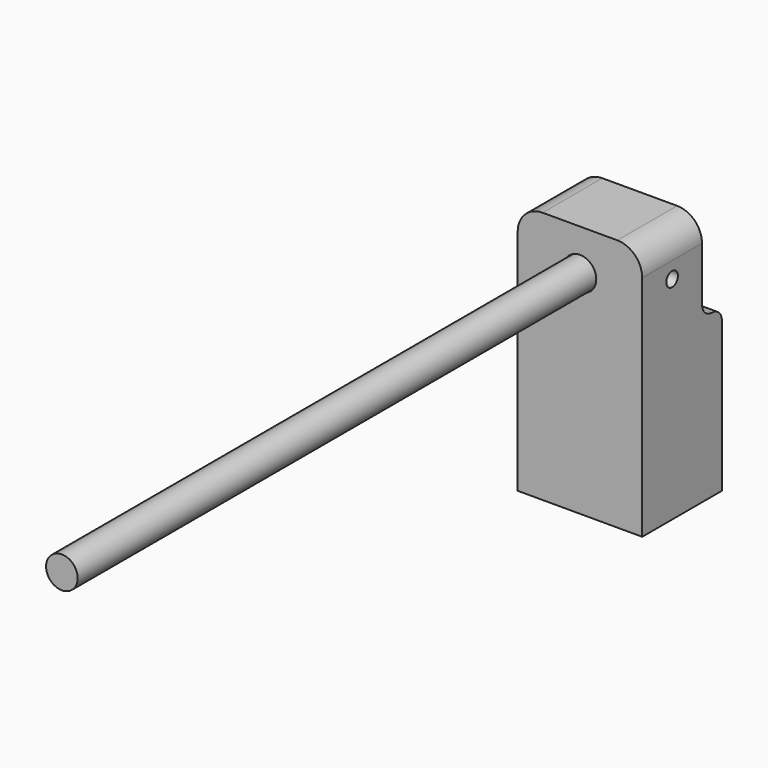
from build123d import *

# Parameters (mm, degrees)
F0_W      = 50
F0_H      = 101.55
F0_R      = 6.55
F1_DEPTH  = 40
F3_R      = 2.9
F4_DEPTH  = 50.001
F5_R      = 2.9
F6_DEPTH  = 25
F7_SIZE   = 2.9
F8_R      = 10
F9_W      = 50
F9_H      = 36.55
F9_R      = 6.55
F10_DEPTH = 10
F11_R     = 4.99999
F0_R_2    = 6.35
F12_DEPTH = 300


# Not quite as in the source:
# - a fillet or chamfer is up to 0.001 mm smaller than in the source, because OpenCascade refuses the exact size


with BuildPart() as f1:
    # F0 (on Front) → F1 (new body)
    with BuildSketch(Plane.XZ):
        with Locations((25, 50.775)):
            Rectangle(F0_W, F0_H)
        with Locations((25, 85)):
            Circle(F0_R, mode=Mode.SUBTRACT)
    extrude(amount=F1_DEPTH)

    # F3 (on face) → F4 (cut, through all)
    with BuildSketch(Plane(origin=(0, 0, 0), x_dir=(0, -1, 0), z_dir=(-1, 0, 0))):
        with Locations((25, 85)):
            Circle(F3_R)
    extrude(amount=-F4_DEPTH, mode=Mode.SUBTRACT)

    # F5 (on face) → F6 (cut)
    with BuildSketch(Plane(origin=(0, 0, 0), x_dir=(1, 0, 0), z_dir=(0, 0, -1))):
        with Locations((10, 25)):
            Circle(F5_R)
        with Locations((25, 25)):
            Circle(F5_R)
        with Locations((40, 25)):
            Circle(F5_R)
    extrude(amount=-F6_DEPTH, mode=Mode.SUBTRACT)

    # F7
    f7_edges = [f1.edges().sort_by_distance(p)[0] for p in [
        (22.1, -25, 25),
        (7.1, -25, 25),
        (37.1, -25, 25),
    ]]
    chamfer(f7_edges, length=F7_SIZE)

    # F8
    f8_edges = [f1.edges().sort_by_distance(p)[0] for p in [
        (50, -20, 101.55),
        (0, -20, 101.55),
    ]]
    fillet(f8_edges, radius=F8_R)

    # F9 (on face) → F10 (cut)
    with BuildSketch(Plane.XZ):
        with Locations((25, 83.275)):
            Rectangle(F9_W, F9_H)
        with Locations((25, 85)):
            Circle(F9_R, mode=Mode.SUBTRACT)
    extrude(amount=F10_DEPTH, mode=Mode.SUBTRACT)

    # F11 (radius 5 in the source; OpenCascade refuses exactly that, so slightly less here)
    f11_edges = [f1.edges().sort_by_distance(p)[0] for p in [
        (25, -10, 65),
        (25, 0, 65),
    ]]
    fillet(f11_edges, radius=F11_R)


with BuildPart() as f12:
    # F0 (on Front) → F12 (new body)
    with BuildSketch(Plane.XZ):
        with Locations((25, 85)):
            Circle(F0_R_2)
    extrude(amount=F12_DEPTH)


solid = Compound([f1.part, f12.part])
